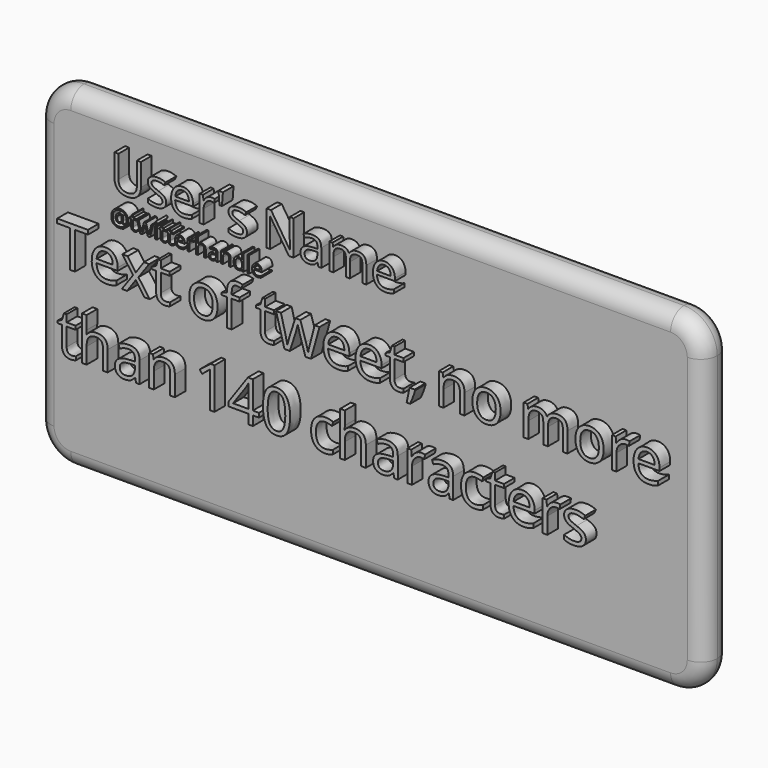
from build123d import *

# Parameters (mm, degrees)
F0_W           = 127
F0_H           = 63.5
F1_DEPTH       = 6.35
F2_R           = 6.35
F3_R           = 3.17246
F5_DEPTH       = 5.08
F5_FACE_R      = 6.35
F7_DEPTH       = 1.27
F8_TEXT_SIZE   = 9.2276904023
F8_TEXT_SIZE_2 = 4.0612787095
F8_TEXT_SIZE_3 = 10.9460675102
F9_DEPTH       = 2.54


# Not quite as in the source:
# - Text() gives the source's letters only with a copy of the font that has no kerning and outlines rounded to 1/6400 em; it was checked with that copy


with BuildPart() as f1:
    # F0 (on Front) → F1 (new body)
    with BuildSketch(Plane.XZ):
        with Locations((-63.5, 31.75)):
            Rectangle(F0_W, F0_H)
    extrude(amount=F1_DEPTH)

    # F2
    f2_edges = [f1.edges().sort_by_distance(p)[0] for p in [
        (-127, -3.175, 63.5),
        (0, -3.175, 63.5),
        (-127, -3.175, 0),
        (0, -3.175, 0),
    ]]
    fillet(f2_edges, radius=F2_R)

    # F3
    f3_edges = [f1.edges().sort_by_distance(p)[0] for p in [
        (-63.5, -6.35, 63.5),
        (-63.5, 0, 63.5),
    ]]
    fillet(f3_edges, radius=F3_R)

    # F4 (on face) → F5 (cut)
    with BuildSketch(Plane(origin=(0, 0, 0), x_dir=(-1, 0, 0), z_dir=(0, 1, 0))):
        with BuildLine():
            Line((20.6529604435, 47.62246), (33.3529604435, 47.62246))
            ThreePointArc((33.3529604435, 47.62246), (27.0029604435, 53.97246), (20.6529604435, 47.62246))
        make_face()
        with BuildLine():
            ThreePointArc((20.6529604435, 47.62246), (27.0029604435, 41.27246), (33.3529604435, 47.62246))
            Line((33.3529604435, 47.62246), (20.6529604435, 47.62246))
        make_face()
        with BuildLine():
            ThreePointArc((101.506557858, 47.62246), (95.156557858, 53.97246), (88.806557858, 47.62246))
            Line((88.806557858, 47.62246), (101.506557858, 47.62246))
        make_face()
        with BuildLine():
            Line((101.506557858, 47.62246), (88.806557858, 47.62246))
            ThreePointArc((88.806557858, 47.62246), (95.156557858, 41.27246), (101.506557858, 47.62246))
        make_face()
    extrude(amount=-F5_DEPTH, mode=Mode.SUBTRACT)

    # F6 (on face) + F5_face (on face) → F7 (join)
    with BuildSketch(Plane(origin=(0, 0, 0), x_dir=(-1, 0, 0), z_dir=(0, 1, 0))):
        with BuildLine():
            ThreePointArc((32.8228315761, 50.16246), (27.0029604435, 53.97246), (21.1830893109, 50.16246))
            Line((21.1830893109, 50.16246), (32.8228315761, 50.16246))
        make_face()
        with BuildLine():
            ThreePointArc((100.9764289906, 50.16246), (95.156557858, 53.97246), (89.3366867254, 50.16246))
            Line((89.3366867254, 50.16246), (100.9764289906, 50.16246))
        make_face()
    with BuildSketch(Plane(origin=(-95.156557858, -5.08, 47.62246), x_dir=(-1, 0, 0), z_dir=(0, 1, 0))):
        Circle(F5_FACE_R)
    extrude(amount=-F7_DEPTH)

    # F8 (on face) → F9 (join)
    with BuildSketch(Plane.XZ.offset(6.35)):
        with Locations((-111.12754, 51.1436029104)):
            Text("User's Name", F8_TEXT_SIZE, font='Open Sans', text_align=(TextAlign.LEFT, TextAlign.BOTTOM))
        with Locations((-111.12754, 45.6794822395)):
            Text('@twitterhandle', F8_TEXT_SIZE_2, font='Open Sans', text_align=(TextAlign.LEFT, TextAlign.BOTTOM))
        with Locations((-121.28754, 35.2583136322)):
            Text('Text of tweet, no more', F8_TEXT_SIZE_3, font='Open Sans', text_align=(TextAlign.LEFT, TextAlign.BOTTOM))
        with Locations((-121.28754, 20.3716618183)):
            Text('than 140 characters', F8_TEXT_SIZE_3, font='Open Sans', text_align=(TextAlign.LEFT, TextAlign.BOTTOM))
    extrude(amount=F9_DEPTH)


solid = f1.part
